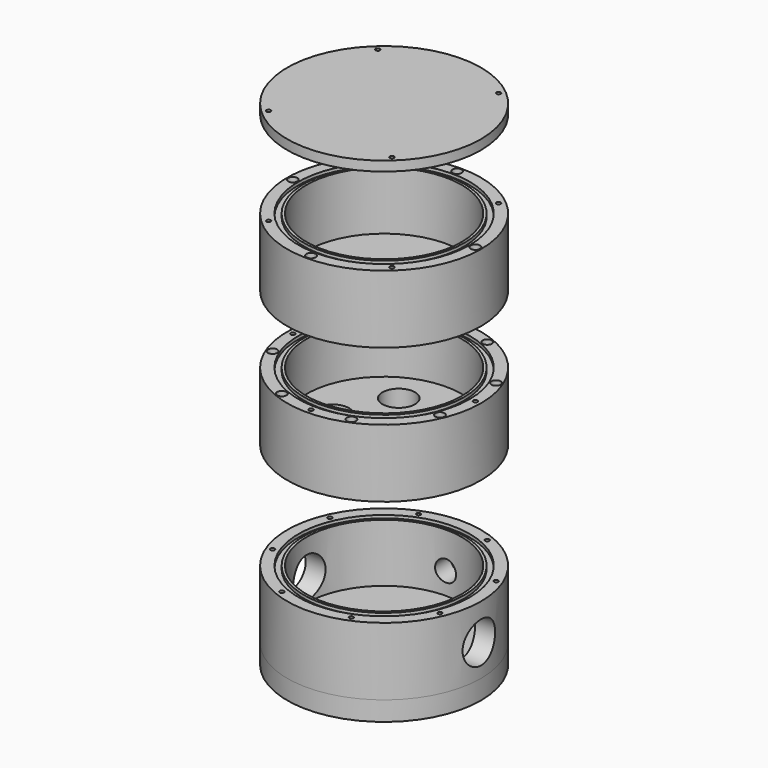
from build123d import *

# Parameters (mm, degrees)
F0_R      = 63.5
F0_R_2    = 50.8
F1_DEPTH  = 44.45
F2_DEPTH  = 6.35
F3_R      = 63.5
F3_R_2    = 50.8
F4_DEPTH  = 25.4
F9_D      = 26.67
F9_DEPTH  = 20.32
F9_TIP    = 8.0124763547
F10_D     = 26.67
F10_DEPTH = 19.05
F10_TIP   = 8.0124763547
F12_R     = 63.5
F12_R_2   = 3.048
F12_R_3   = 50.8
F13_DEPTH = 44.45
F14_R     = 50.8
F15_DEPTH = 12.7
F17_D     = 26.67
F22_D     = 13.716
F22_DEPTH = 15.4178
F22_TIP   = 4.1207021253
F25_R     = 63.5
F26_DEPTH = 6.35
F27_D     = 2.794
F28_D     = 2.794
F19_R     = 63.5
F19_R_2   = 50.8
F29_DEPTH = 44.45
F23_R     = 50.8
F30_DEPTH = 6.35
F33_D     = 2.794
F34_D     = 2.794
F35_D     = 2.794
F36_D     = 2.794
F37_D     = 2.794
F38_D     = 2.794
F39_D     = 2.794
F40_D     = 2.794
F41_R     = 56.1594
F41_R_2   = 52.4764
F42_DEPTH = 2.032
F44_R     = 56.1594
F44_R_2   = 52.4764
F45_DEPTH = 2.032
F47_R     = 56.1594
F47_R_2   = 52.4764
F48_DEPTH = 2.032
F49_D     = 2.794
F50_D     = 6.096
F51_D     = 2.794
F52_D     = 6.096
F53_D     = 6.096
F54_D     = 6.096
F55_D     = 2.794
F56_D     = 2.794
F57_D     = 2.794
F58_D     = 2.794
F59_D     = 2.794
F60_D     = 2.794
F61_D     = 2.794
F62_D     = 2.794
F63_D     = 21.336
F64_D     = 21.336
F65_D     = 13.716
F66_DEPTH = 12.7


with BuildPart() as f1:
    # F0 (on Top) → F1 (new body)
    with BuildSketch(Plane.XY):
        Circle(F0_R)
        Circle(F0_R_2, mode=Mode.SUBTRACT)
    extrude(amount=F1_DEPTH)

    # F0 (on Top) → F2 (join)
    with BuildSketch(Plane.XY):
        Circle(F0_R_2)
    extrude(amount=F2_DEPTH)

    # F3 (on Top) → F4 (join)
    with BuildSketch(Plane.XY):
        Circle(F3_R)
        Circle(F3_R_2, mode=Mode.SUBTRACT)
    extrude(amount=F4_DEPTH)

    # F9
    with Locations(Plane.YZ.offset(63.5)):
        with Locations((0, 20.7972154021)):
            Hole(F9_D / 2, depth=F9_DEPTH)
            with Locations((0, 0, -(F9_DEPTH + F9_TIP / 2))):  # 118° drill point
                Cone(0, F9_D / 2, F9_TIP, mode=Mode.SUBTRACT)

    # F10
    with Locations(Plane(origin=(-63.5, 0, 0), x_dir=(0, 1, 0), z_dir=(-1, 0, 0))):
        with Locations((0, -20.7972154021)):
            Hole(F10_D / 2, depth=F10_DEPTH)
            with Locations((0, 0, -(F10_DEPTH + F10_TIP / 2))):  # 118° drill point
                Cone(0, F10_D / 2, F10_TIP, mode=Mode.SUBTRACT)

    # F22
    with Locations(Plane(origin=(0, 63.5, 0), x_dir=(1, 0, 0), z_dir=(0, 1, 0))):
        with Locations((0, -20.7910817116)):
            Hole(F22_D / 2, depth=F22_DEPTH)
            with Locations((0, 0, -(F22_DEPTH + F22_TIP / 2))):  # 118° drill point
                Cone(0, F22_D / 2, F22_TIP, mode=Mode.SUBTRACT)

    # F33 (through all)
    with Locations(Plane.XY.offset(44.45)):
        with Locations((-55.837423015, -21.5242892754)):
            Hole(F33_D / 2)

    # F34 (through all)
    with Locations(Plane.XY.offset(44.45)):
        with Locations((-22.7539731958, -55.3477148721)):
            Hole(F34_D / 2)

    # F35 (through all)
    with Locations(Plane.XY.offset(44.45)):
        with Locations((-54.7935706029, 24.0577941289)):
            Hole(F35_D / 2)

    # F36 (through all)
    with Locations(Plane.XY.offset(44.45)):
        with Locations((-21.9543816141, 55.669722163)):
            Hole(F36_D / 2)

    # F37 (through all)
    with Locations(Plane.XY.offset(44.45)):
        with Locations((23.6277017902, 54.9804014707)):
            Hole(F37_D / 2)

    # F38 (through all)
    with Locations(Plane.XY.offset(44.45)):
        with Locations((55.4959820047, 22.3899267327)):
            Hole(F38_D / 2)

    # F39 (through all)
    with Locations(Plane.XY.offset(44.45)):
        with Locations((55.1655391226, -23.1921566715)):
            Hole(F39_D / 2)

    # F40 (through all)
    with Locations(Plane.XY.offset(44.45)):
        with Locations((22.8281102084, -55.3171783633)):
            Hole(F40_D / 2)

    # F41 (on offset) → F42 (cut)
    with BuildSketch(Plane.XY.offset(44.45)):
        Circle(F41_R)
        Circle(F41_R_2, mode=Mode.SUBTRACT)
    extrude(amount=-F42_DEPTH, mode=Mode.SUBTRACT)

    # F0 (on Top) → F66 (join)
    with BuildSketch(Plane.XY):
        Circle(F0_R)
        Circle(F0_R_2, mode=Mode.SUBTRACT)
        Circle(F0_R_2)
    extrude(amount=-F66_DEPTH)


with BuildPart() as f13:
    # F12 (on offset) → F13 (new body)
    with BuildSketch(Plane.XY.offset(114.3)):
        Circle(F12_R)
        with Locations((-22.7539731958, -55.3477148721)):
            Circle(F12_R_2, mode=Mode.SUBTRACT)
        with Locations((-55.837423015, -21.5242892754)):
            Circle(F12_R_2, mode=Mode.SUBTRACT)
        with Locations((22.8281102084, -55.3171783633)):
            Circle(F12_R_2, mode=Mode.SUBTRACT)
        with Locations((55.1655391226, -23.1921566715)):
            Circle(F12_R_2, mode=Mode.SUBTRACT)
        with Locations((-54.7935706029, 24.0577941289)):
            Circle(F12_R_2, mode=Mode.SUBTRACT)
        with Locations((-21.9543816141, 55.669722163)):
            Circle(F12_R_2, mode=Mode.SUBTRACT)
        Circle(F12_R_3, mode=Mode.SUBTRACT)
        with Locations((55.4959820047, 22.3899267327)):
            Circle(F12_R_2, mode=Mode.SUBTRACT)
        with Locations((23.6277017902, 54.9804014707)):
            Circle(F12_R_2, mode=Mode.SUBTRACT)
    extrude(amount=F13_DEPTH)

    # F14 (on offset) → F15 (join)
    with BuildSketch(Plane.XY.offset(114.3)):
        Circle(F14_R)
    extrude(amount=F15_DEPTH)

    # F17 (through all)
    with Locations(Plane(origin=(0, 0, 114.3), x_dir=(1, 0, 0), z_dir=(0, 0, -1))):
        with Locations((11.686825238, 25.3783710245)):
            Hole(F17_D / 2)

    # F27 (through all)
    with Locations(Plane.XY.offset(203.2)):
        with Locations((0, 59.8424)):
            Hole(F27_D / 2)

    # F44 (on offset) → F45 (cut)
    with BuildSketch(Plane.XY.offset(158.75)):
        Circle(F44_R)
        Circle(F44_R_2, mode=Mode.SUBTRACT)
    extrude(amount=-F45_DEPTH, mode=Mode.SUBTRACT)

    # F49 (through all)
    with Locations(Plane.XY.offset(203.2)):
        with Locations((0, -59.8424)):
            Hole(F49_D / 2)

    # F51 (through all)
    with Locations(Plane.XY.offset(203.2)):
        with Locations((59.8424, 0)):
            Hole(F51_D / 2)

    # F55 (through all)
    with Locations(Plane.XY.offset(203.2)):
        with Locations((-59.8424, 0)):
            Hole(F55_D / 2)

    # F63 (through all)
    with Locations(Plane(origin=(0, 0, 114.3), x_dir=(1, 0, 0), z_dir=(0, 0, -1))):
        with Locations((-26.413174762, 9.1097639373)):
            Hole(F63_D / 2)

    # F64 (through all)
    with Locations(Plane(origin=(0, 0, 114.3), x_dir=(1, 0, 0), z_dir=(0, 0, -1))):
        with Locations((-10.942729788, -25.7079805661)):
            Hole(F64_D / 2)

    # F65 (through all)
    with Locations(Plane(origin=(0, 0, 114.3), x_dir=(1, 0, 0), z_dir=(0, 0, -1))):
        with Locations((24.8757664447, -12.7216289755)):
            Hole(F65_D / 2)


with BuildPart() as f26:
    # F25 (on offset) → F26 (new body)
    with BuildSketch(Plane.XY.offset(304.8)):
        Circle(F25_R)
    extrude(amount=F26_DEPTH)

    # F28 (through all)
    with Locations(Plane(origin=(0, 0, 304.8), x_dir=(1, 0, 0), z_dir=(0, 0, -1))):
        with Locations((-39.7570301478, -44.5227431076)):
            Hole(F28_D / 2)

    # F57 (through all)
    with Locations(Plane(origin=(0, 0, 304.8), x_dir=(1, 0, 0), z_dir=(0, 0, -1))):
        with Locations((-40.9610582496, 43.4175978962)):
            Hole(F57_D / 2)

    # F60 (through all)
    with Locations(Plane(origin=(0, 0, 304.8), x_dir=(1, 0, 0), z_dir=(0, 0, -1))):
        with Locations((40.3384601317, 43.9966445789)):
            Hole(F60_D / 2)

    # F61 (through all)
    with Locations(Plane(origin=(0, 0, 304.8), x_dir=(1, 0, 0), z_dir=(0, 0, -1))):
        with Locations((38.6580461216, -45.4802327397)):
            Hole(F61_D / 2)


with BuildPart() as f29:
    # F19 (on offset) → F29 (new body)
    with BuildSketch(Plane.XY.offset(203.2)):
        Circle(F19_R)
        Circle(F19_R_2, mode=Mode.SUBTRACT)
    extrude(amount=F29_DEPTH)

    # F23 (on offset) → F30 (join)
    with BuildSketch(Plane.XY.offset(203.2)):
        Circle(F23_R)
    extrude(amount=F30_DEPTH)

    # F47 (on offset) → F48 (cut)
    with BuildSketch(Plane.XY.offset(247.65)):
        Circle(F47_R)
        Circle(F47_R_2, mode=Mode.SUBTRACT)
    extrude(amount=-F48_DEPTH, mode=Mode.SUBTRACT)

    # F50 (through all)
    with Locations(Plane(origin=(0, 0, 203.2), x_dir=(1, 0, 0), z_dir=(0, 0, -1))):
        with Locations((0, 59.8424)):
            Hole(F50_D / 2)

    # F52 (through all)
    with Locations(Plane(origin=(0, 0, 203.2), x_dir=(1, 0, 0), z_dir=(0, 0, -1))):
        with Locations((59.8424, 0)):
            Hole(F52_D / 2)

    # F53 (through all)
    with Locations(Plane(origin=(0, 0, 203.2), x_dir=(1, 0, 0), z_dir=(0, 0, -1))):
        with Locations((0, -59.8424)):
            Hole(F53_D / 2)

    # F54 (through all)
    with Locations(Plane(origin=(0, 0, 203.2), x_dir=(1, 0, 0), z_dir=(0, 0, -1))):
        with Locations((-59.8424, 0)):
            Hole(F54_D / 2)

    # F56 (through all)
    with Locations(Plane.XY.offset(304.8)):
        with Locations((-39.7570301478, 44.5227431076)):
            Hole(F56_D / 2)

    # F58 (through all)
    with Locations(Plane.XY.offset(304.8)):
        with Locations((-40.9610582496, -43.4175978962)):
            Hole(F58_D / 2)

    # F59 (through all)
    with Locations(Plane.XY.offset(304.8)):
        with Locations((40.3384601317, -43.9966445789)):
            Hole(F59_D / 2)

    # F62 (through all)
    with Locations(Plane.XY.offset(304.8)):
        with Locations((38.6580461216, 45.4802327397)):
            Hole(F62_D / 2)


solid = Compound([f1.part, f13.part, f26.part, f29.part])
